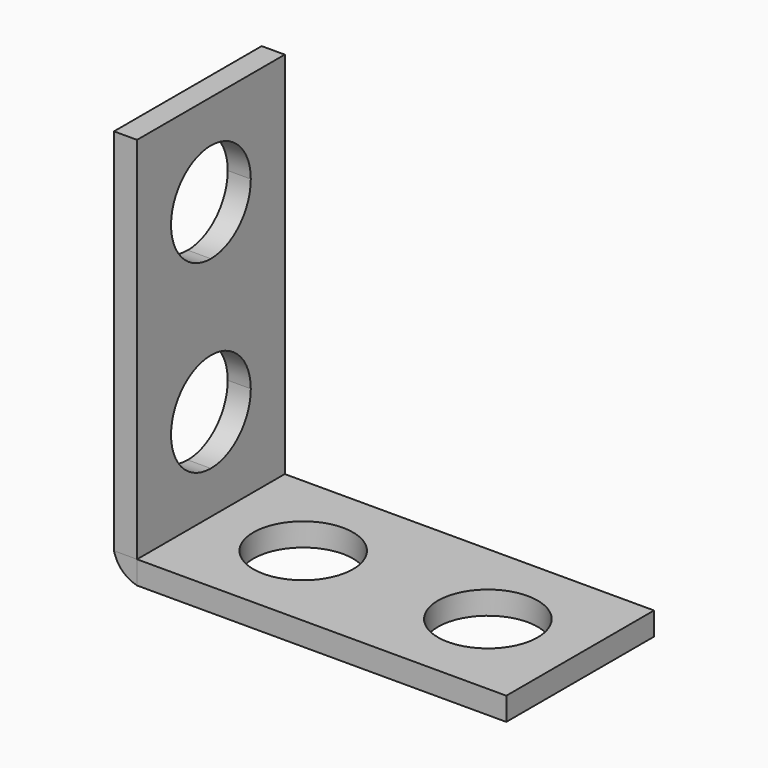
from build123d import *

# Parameters (mm, degrees)
F1_DEPTH    = 1.5875
F3_DEPTH    = 1.5875
F4_W        = 1.5875
F4_H        = 1.5875
F5_DEPTH    = 12.7
F6_T1_DEPTH = 20.6375


# Not quite as in the source:
# - a fillet or chamfer that OpenCascade refuses, or shapes differently, is made with other operations: its cross-section is extruded or revolved along the edge and cut away or added


with BuildPart() as f1:
    # F0 (on Right) → F1 (new body)
    with BuildSketch(Plane.YZ):
        with BuildLine():
            Line((0, 25.4), (0, 0))
            Line((0, 0), (6.35, 0))
            Line((6.35, 0), (6.35, 2.921))
            ThreePointArc((6.35, 2.921), (2.921, 6.35), (6.35, 9.779))
            Line((6.35, 9.779), (6.35, 12.7))
            Line((6.35, 12.7), (6.35, 15.621))
            ThreePointArc((6.35, 15.621), (2.921, 19.05), (6.35, 22.479))
            Line((6.35, 22.479), (6.35, 25.4))
            Line((6.35, 25.4), (0, 25.4))
        make_face()
        with BuildLine():
            Line((6.35, 2.921), (6.35, 0))
            Line((6.35, 0), (12.7, 0))
            Line((12.7, 0), (12.7, 25.4))
            Line((12.7, 25.4), (6.35, 25.4))
            Line((6.35, 25.4), (6.35, 22.479))
            ThreePointArc((6.35, 22.479), (8.7746691527, 21.4746691527), (9.779, 19.05))
            ThreePointArc((9.779, 19.05), (8.7746691527, 16.6253308473), (6.35, 15.621))
            Line((6.35, 15.621), (6.35, 12.7))
            Line((6.35, 12.7), (6.35, 9.779))
            ThreePointArc((6.35, 9.779), (8.7746691527, 8.7746691527), (9.779, 6.35))
            ThreePointArc((9.779, 6.35), (8.7746691527, 3.9253308473), (6.35, 2.921))
        make_face()
    extrude(amount=F1_DEPTH)


with BuildPart() as f3:
    # F2 (on Top) → F3 (new body)
    with BuildSketch(Plane.XY):
        with BuildLine():
            Line((1.5875, 6.35), (1.5875, 0))
            Line((1.5875, 0), (26.9875, 0))
            Line((26.9875, 0), (26.9875, 6.35))
            Line((26.9875, 6.35), (24.0665, 6.35))
            ThreePointArc((24.0665, 6.35), (20.6375, 2.921), (17.2085, 6.35))
            Line((17.2085, 6.35), (14.2875, 6.35))
            Line((14.2875, 6.35), (11.3665, 6.35))
            ThreePointArc((11.3665, 6.35), (7.9375, 2.921), (4.5085, 6.35))
            Line((4.5085, 6.35), (1.5875, 6.35))
        make_face()
        with BuildLine():
            Line((1.5875, 12.7), (1.5875, 6.35))
            Line((1.5875, 6.35), (4.5085, 6.35))
            ThreePointArc((4.5085, 6.35), (7.9375, 9.779), (11.3665, 6.35))
            Line((11.3665, 6.35), (14.2875, 6.35))
            Line((14.2875, 6.35), (17.2085, 6.35))
            ThreePointArc((17.2085, 6.35), (20.6375, 9.779), (24.0665, 6.35))
            Line((24.0665, 6.35), (26.9875, 6.35))
            Line((26.9875, 6.35), (26.9875, 12.7))
            Line((26.9875, 12.7), (1.5875, 12.7))
        make_face()
    extrude(amount=-F3_DEPTH)


with BuildPart() as f5:
    # F4 (on Front) → F5 (new body, through all)
    with BuildSketch(Plane.XZ):
        with Locations((0.79375, -0.79375)):
            Rectangle(F4_W, F4_H)
    extrude(amount=-F5_DEPTH)

    # F6: fillet of radius 2.2606 on 1 edges, made by hand

    # F6_s2 → F6_t1 (cut)
    with BuildSketch(Plane.XZ.offset(-16.66875)):
        with BuildLine():
            add(Edge.make_bspline(
                [(0, 0), (0.3396631777, -1.2478368223), (1.5875, -1.5875)],
                knots=[0, 0, 0, 1, 1, 1], degree=2, weights=[1, 1, 1]))
            Line((1.5875, -1.5875), (0, -1.5875))
            Line((0, -1.5875), (0, 0))
        make_face()
    extrude(amount=F6_T1_DEPTH, mode=Mode.SUBTRACT)


solid = Compound([f1.part, f3.part, f5.part])
